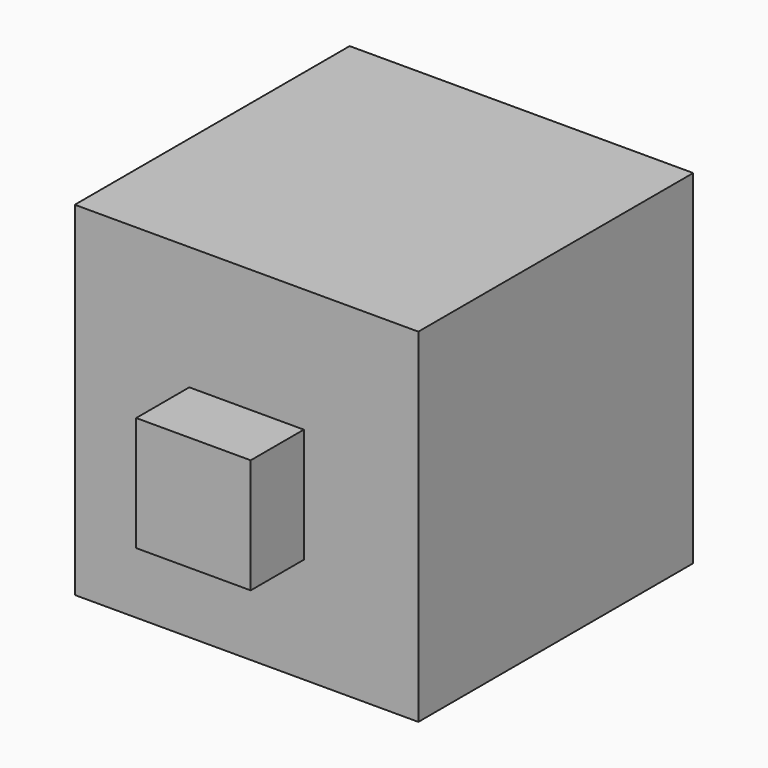
from build123d import *

# Parameters (mm, degrees)
F0_W     = 76.2
F0_H     = 76.2
F1_DEPTH = 25.4
F2_DEPTH = 76.2
F3_W     = 25.4
F3_H     = 25.4
F4_DEPTH = 14.732


# Not quite as in the source:
# - the program builds the solid bodies; features that only make, move or delete a surface that nothing else refers to are left out


with BuildPart() as f1:
    # F0 (on Front) → F1 (new body)
    with BuildSketch(Plane.XZ):
        with Locations((-38.1, 42.3055109791)):
            Rectangle(F0_W, F0_H)
    extrude(amount=F1_DEPTH)

    # F0 (on Front) → F2 (join)
    with BuildSketch(Plane.XZ):
        with Locations((-38.1, 42.3055109791)):
            Rectangle(F0_W, F0_H)
    extrude(amount=F2_DEPTH)

    # F3 (on face) → F4 (join)
    with BuildSketch(Plane.XZ.offset(76.2)):
        with Locations((-38.1, 40.3138278052)):
            Rectangle(F3_W, F3_H)
    extrude(amount=F4_DEPTH)


solid = f1.part
